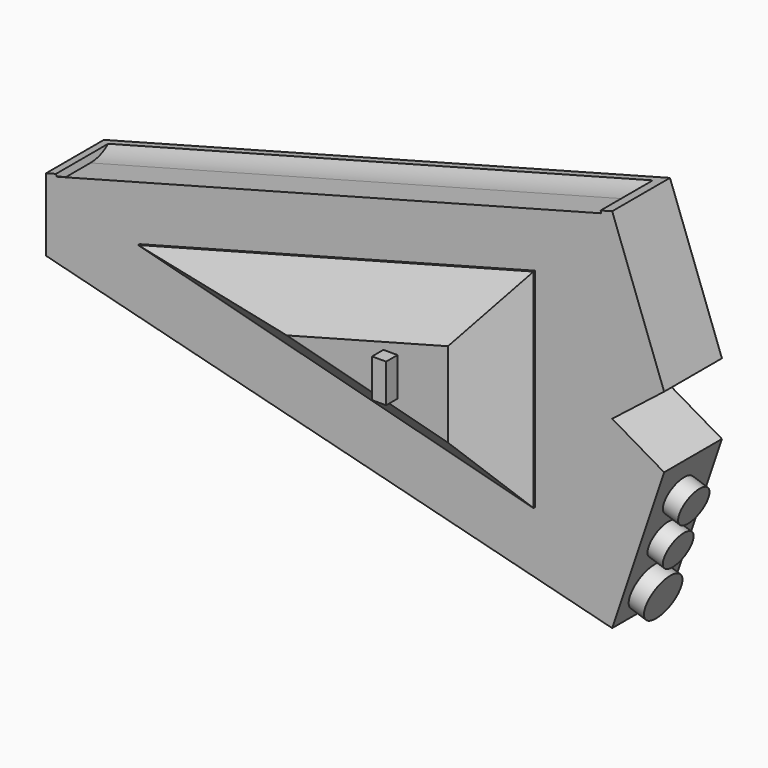
from build123d import *

# Parameters (mm, degrees)
F1_DEPTH     = 7.6
F3_DEPTH     = 5.2
F4_R         = 1.8844883856
F4_R_2       = 1.9205503988
F4_R_3       = 2.3505118907
F5_DEPTH     = 1.7
F6_SIZE      = 5
F7_W         = 1.4806352556
F7_H         = 4.0441937745
F8_DEPTH     = 1.5
F9_W         = 59.2752462253
F9_H         = 5.8640984353
F10_DEPTH    = 0.7
F11_T1_DEPTH = 59.2752462253
F11_T3_DEPTH = 59.2752462253


# Not quite as in the source:
# - a fillet or chamfer that OpenCascade refuses, or shapes differently, is made with other operations: its cross-section is extruded or revolved along the edge and cut away or added


with BuildPart() as f1:
    # F0 (on Front) → F1 (new body)
    with BuildSketch(Plane.XZ):
        Polygon((0, 19.2095376551), (-59.5404654741, 3.3684971277), (-59.5404654741, -4.2789019644), (0, -19.391618669), (5.4624280892, -3.1864163466), (0, 0), (5.4624280892, 4.2789019644), align=None)
    extrude(amount=F1_DEPTH)

    # F2 (on face) → F3 (join)
    with BuildSketch(Plane.XZ.offset(7.6)):
        Polygon((-8.1104228631, 11.0672699008), (-49.7080944479, 0), (-8.1104228631, -10.8338156715), align=None)
    extrude(amount=F3_DEPTH)

    # F4 (on face) → F5 (join)
    with BuildSketch(Plane(origin=(5.8695867149, 0, -1.978512499), x_dir=(0, 1, 0), z_dir=(0.9476131807, 0, -0.3194201932))):
        with Locations((-4.2056068778, -10.1775936782)):
            Circle(F4_R)
        with Locations((-4.05138731, -5.432640668)):
            Circle(F4_R_2)
        with Locations((-4.1012428701, -15.386570245)):
            Circle(F4_R_3)
    extrude(amount=F5_DEPTH)

    # F6
    f6_edges = [f1.edges().sort_by_distance(p)[0] for p in [
        (-28.909259, -12.8, 5.533635),
        (-28.909259, -12.8, -5.416908),
        (-8.110423, -12.8, 0.116727),
    ]]
    chamfer(f6_edges, length=F6_SIZE)

    # F7 (on face) → F8 (join)
    with BuildSketch(Plane.XZ.offset(12.8)):
        with Locations((-19.157294184, 0)):
            Rectangle(F7_W, F7_H)
    extrude(amount=F8_DEPTH)

    # F9 (on face) → F10 (cut)
    with BuildSketch(Plane(origin=(-4.7729402647, 0, 17.9396728738), x_dir=(0.9663819367, 0, 0.2571107784), z_dir=(-0.2571107784, 0, 0.9663819367))):
        with Locations((-25.96012922, -3.6729333224)):
            Rectangle(F9_W, F9_H)
    extrude(amount=-F10_DEPTH, mode=Mode.SUBTRACT)

    # F11: fillet of radius 5 on 2 edges, made by hand

    # F11_s2 → F11_t1 (join)
    with BuildSketch(Plane(origin=(3.5538636702, 0, 0.9455233173), x_dir=(0, 1, 0), z_dir=(-0.9663819367, 0, -0.2571107784))):
        with BuildLine():
            ThreePointArc((-0.7408841047, -18.5637502027), (-1.9694786136, -18.0419248222), (-3.2923542692, -17.8637502027))
            Line((-3.2923542692, -17.8637502027), (-0.7408841047, -17.8637502027))
            Line((-0.7408841047, -17.8637502027), (-0.7408841047, -18.5637502027))
        make_face()
    extrude(amount=F11_T1_DEPTH)

    # F11_s4 → F11_t3 (cut)
    with BuildSketch(Plane(origin=(-53.7286635768, 0, -14.2947813798), x_dir=(0, 1, 0), z_dir=(0.9663819367, 0, 0.2571107784))):
        with BuildLine():
            ThreePointArc((-9.1564527044, 18.5637502027), (-7.8335770489, 18.3855755832), (-6.60498254, 17.8637502027))
            Line((-6.60498254, 17.8637502027), (-6.60498254, 18.5637502027))
            Line((-6.60498254, 18.5637502027), (-9.1564527044, 18.5637502027))
        make_face()
    extrude(amount=F11_T3_DEPTH, mode=Mode.SUBTRACT)


solid = f1.part
